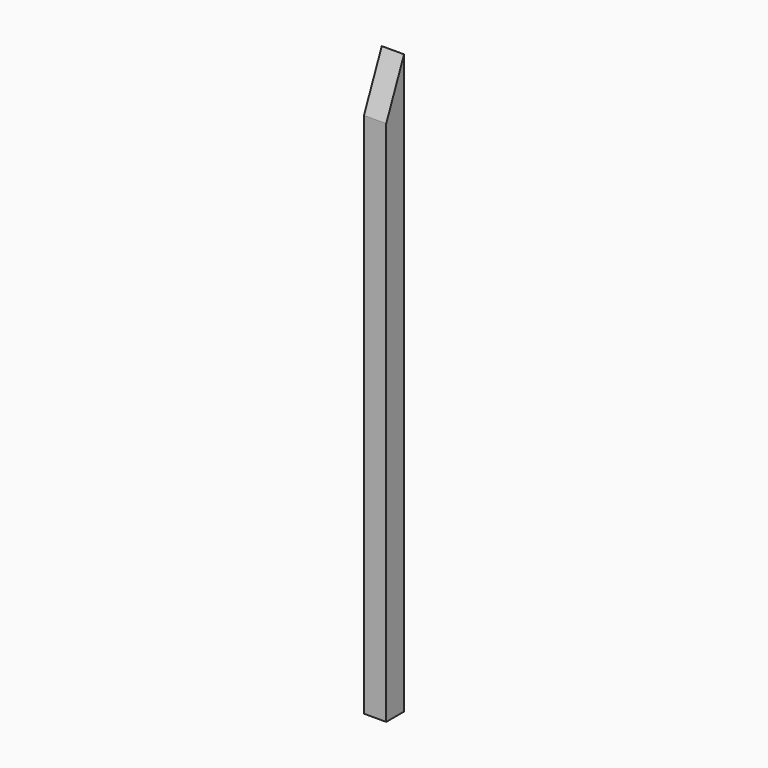
from build123d import *

# Parameters (mm, degrees)
F1_DEPTH = 3.175


# Not quite as in the source:
# - a feature names something its author has since deleted; it is built from what else it names


with BuildPart() as f1:
    # F0 (on Right) → F1 (new body)
    with BuildSketch(Plane.YZ):
        Polygon((3.175, 0), (3.175, 82.55), (0, 75.1416666667), (0, 0), align=None)
    extrude(amount=F1_DEPTH)


solid = f1.part
